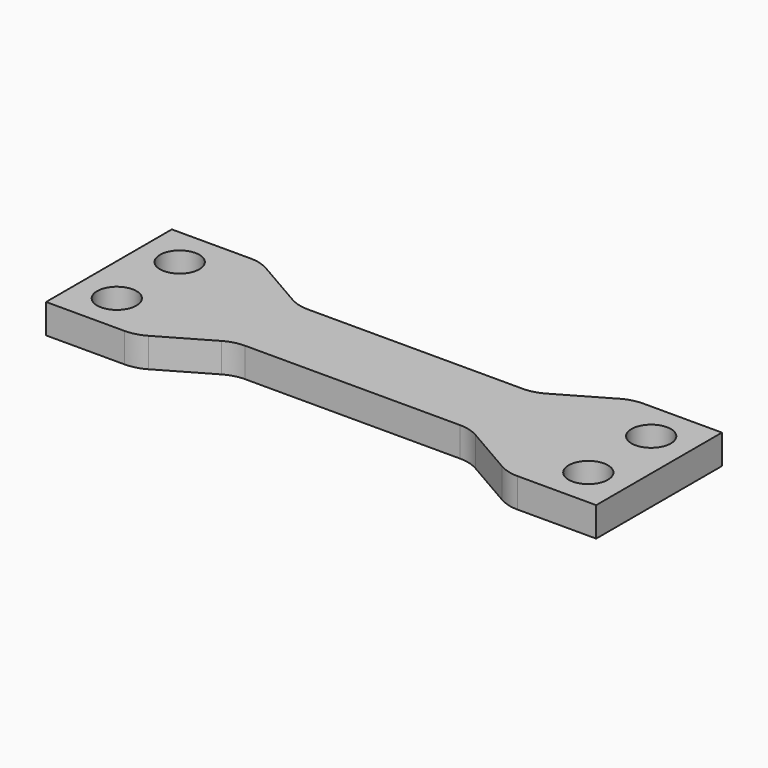
from build123d import *

# Parameters (mm, degrees)
F0_R     = 1
F1_DEPTH = 1.5


# Not quite as in the source:
# - ends of sketch curves that miss each other by under 0.0002 mm in the source are joined


with BuildPart() as f1:
    # F0 (on Top) → F1 (new body)
    with BuildSketch(Plane.XY):
        with BuildLine():
            Line((6.464165, -2.26795), (9.000064, -3.732051))
            ThreePointArc((9.000064, -3.732051), (9.4824259563, -3.931851665), (10.000064, -4))
            Line((10.000064, -4), (14.000064, -4))
            Line((14.000064, -4), (14.000064, 4))
            Line((14.000064, 4), (10.000064, 4))
            ThreePointArc((10.000064, 4), (9.4824257148, 3.9318516003), (9.0000636503, 3.7320506057))
            Line((9.0000636503, 3.7320506057), (6.464165, 2.267949))
            ThreePointArc((6.464165, 2.267949), (5.9817417072, 2.0681319009), (5.464038, 2.000000004))
            Line((5.464038, 2.000000004), (-5.464038, 2))
            ThreePointArc((-5.464038, 2), (-5.9817422242, 2.0681317715), (-6.4641659167, 2.2679491443))
            Line((-6.4641659167, 2.2679491443), (-9.000064, 3.73205))
            ThreePointArc((-9.000064, 3.73205), (-9.4824257148, 3.9318516003), (-10.000064, 4))
            Line((-10.000064, 4), (-14.000064, 4))
            Line((-14.000064, 4), (-14.000064, -4))
            Line((-14.000064, -4), (-10.000064, -4))
            ThreePointArc((-10.000064, -4), (-9.4824259563, -3.931851665), (-9.0000640833, -3.7320508557))
            Line((-9.0000640833, -3.7320508557), (-6.464166, -2.26795))
            ThreePointArc((-6.464166, -2.26795), (-5.9817424657, -2.0681318362), (-5.464038, -2.0000000041))
            Line((-5.464038, -2.0000000041), (5.464038, -2))
            ThreePointArc((5.464038, -2), (5.9817419487, -2.0681319656), (6.464165, -2.26795))
        make_face()
        with Locations((-12.000064, -2)):
            Circle(F0_R, mode=Mode.SUBTRACT)
        with Locations((12.000064, -2)):
            Circle(F0_R, mode=Mode.SUBTRACT)
        with Locations((-12.000064, 2)):
            Circle(F0_R, mode=Mode.SUBTRACT)
        with Locations((12.000064, 2)):
            Circle(F0_R, mode=Mode.SUBTRACT)
    extrude(amount=F1_DEPTH)


solid = f1.part
